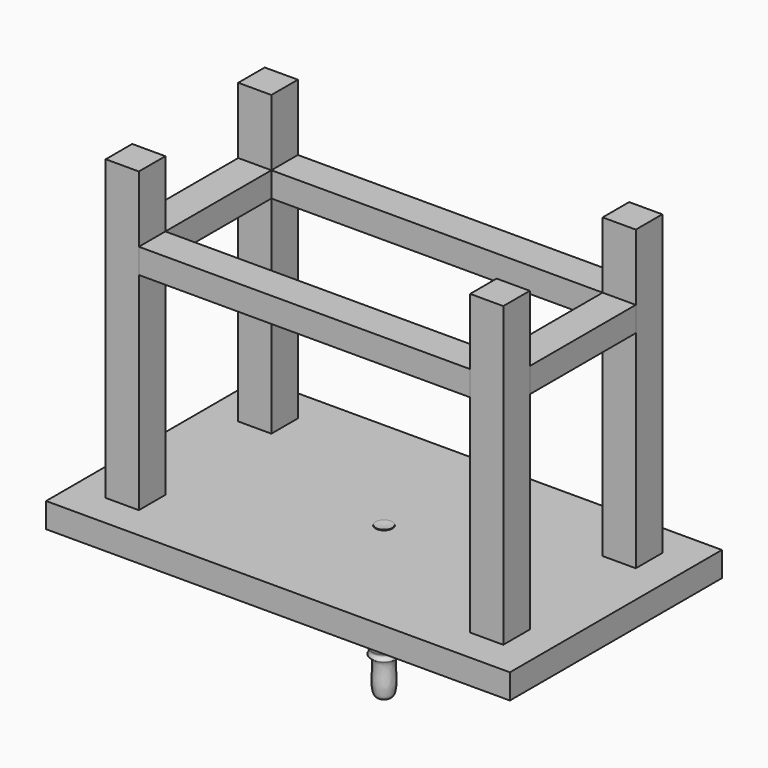
from build123d import *

# Parameters (mm, degrees)
F0_W          = 101.6
F0_H          = 101.6
F1_DEPTH      = 914.4
F2_W          = 101.6
F2_H          = 76.2
F3_DEPTH      = 1016
F4_W          = 101.6
F4_H          = 76.2
F5_DEPTH      = 406.4
F6_W          = 1422.4
F6_H          = 76.2
F7_DEPTH      = 406.4
F7_DEPTH_BACK = 406.4


with BuildPart() as f1:
    # F0 (on Top) → F1 (new body)
    with BuildSketch(Plane.XY):
        with Locations((-558.8, 254)):
            Rectangle(F0_W, F0_H)
    extrude(amount=F1_DEPTH)


with BuildPart() as f1b:
    # F0 (on Top) → F1, piece 2 (new body)
    with BuildSketch(Plane.XY):
        with Locations((-558.8, -254)):
            Rectangle(F0_W, F0_H)
    extrude(amount=F1_DEPTH)


with BuildPart() as f1c:
    # F0 (on Top) → F1, piece 3 (new body)
    with BuildSketch(Plane.XY):
        with Locations((558.8, 254)):
            Rectangle(F0_W, F0_H)
    extrude(amount=F1_DEPTH)


with BuildPart() as f1d:
    # F0 (on Top) → F1, piece 4 (new body)
    with BuildSketch(Plane.XY):
        with Locations((558.8, -254)):
            Rectangle(F0_W, F0_H)
    extrude(amount=F1_DEPTH)


with BuildPart() as f3:
    # F2 (on face) → F3 (new body)
    with BuildSketch(Plane.YZ.offset(-508)):
        with Locations((-254, 673.1)):
            Rectangle(F2_W, F2_H)
    extrude(amount=F3_DEPTH)


with BuildPart() as f3b:
    # F2 (on face) → F3, piece 2 (new body)
    with BuildSketch(Plane.YZ.offset(-508)):
        with Locations((254, 673.1)):
            Rectangle(F2_W, F2_H)
    extrude(amount=F3_DEPTH)


with BuildPart() as f5:
    # F4 (on face) → F5 (new body)
    with BuildSketch(Plane(origin=(0, -203.2, 0), x_dir=(-1, 0, 0), z_dir=(0, 1, 0))):
        with Locations((-558.8, 673.1)):
            Rectangle(F4_W, F4_H)
    extrude(amount=F5_DEPTH)


with BuildPart() as f5b:
    # F4 (on face) → F5, piece 2 (new body)
    with BuildSketch(Plane(origin=(0, -203.2, 0), x_dir=(-1, 0, 0), z_dir=(0, 1, 0))):
        with Locations((558.8, 673.1)):
            Rectangle(F4_W, F4_H)
    extrude(amount=F5_DEPTH)


with BuildPart() as f7:
    # F6 (on Front) → F7 (new body, two sides)
    with BuildSketch(Plane.XZ) as f7_sk:
        with Locations((0, -38.1)):
            Rectangle(F6_W, F6_H)
    extrude(amount=-F7_DEPTH)
    extrude(f7_sk.sketch, amount=F7_DEPTH_BACK)

    # F8 (on Right) → F9 (revolve)
    with BuildSketch(Plane.YZ):
        with BuildLine():
            Line((25.4638567567, 1.8187186215), (0, 0))
            Line((0, 0), (0, -454.8777937889))
            add(Edge.make_bspline(
                [(25.4638567567, 1.8187186215), (34.4382523346, -34.7031738143), (56.9012899023, -111.0496230705), (27.0788695893, -207.6950770004), (25.4154335933, -313.8808837767), (45.3355488252, -323.2209863813), (29.4925793524, -334.9241454751), (44.8346681145, -348.3242520498), (22.854328945, -351.7448701182), (34.6092554991, -416.712042373), (25.1374166029, -468.0172844227), (7.2653372186, -458.674717409), (0, -454.8777937889)],
                knots=[0, 0, 0, 0, 0.1664097973, 0.3295758434, 0.484052475, 0.538930427, 0.5944440202, 0.6498239949, 0.7009186508, 0.8259523875, 0.9293484076, 1, 1, 1, 1], degree=3))
        make_face()
    revolve(axis=Axis((0, 0, -227.4388968945), (0, 0, -1)))


solid = Compound([f1.part, f1b.part, f1c.part, f1d.part, f3.part, f3b.part, f5.part, f5b.part, f7.part])
